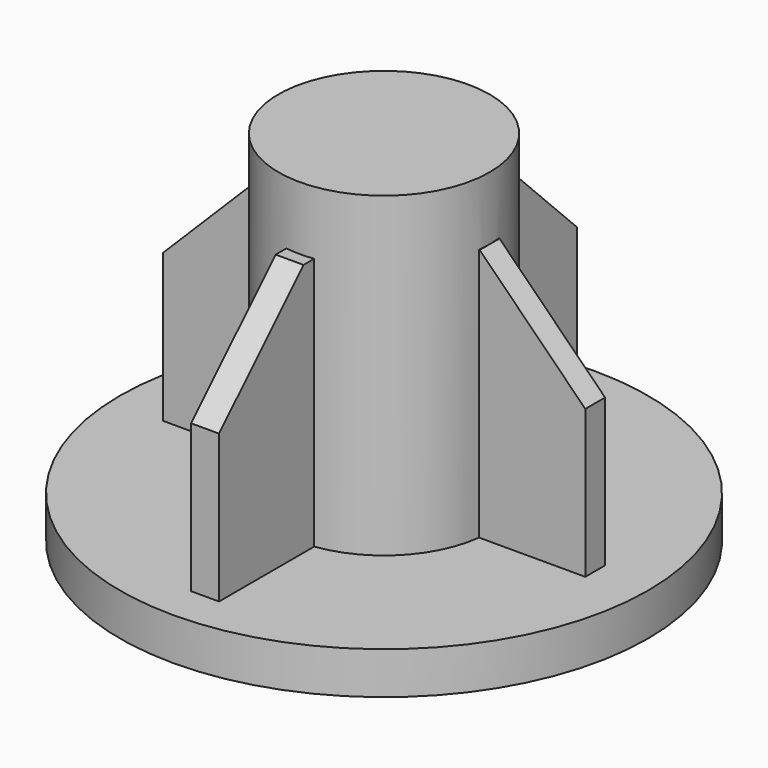
from build123d import *

# Parameters (mm, degrees)
F0_R     = 5
F2_DEPTH = 15
F1_W     = 9.3396854261
F1_H     = 1.1709111985
F1_W_2   = 1.3206291478
F1_H_2   = 10.0037873136
F3_DEPTH = 12
F4_SIZE  = 4.99999
F5_R     = 12.5
F6_DEPTH = 2


# Not quite as in the source:
# - a fillet or chamfer is up to 0.001 mm smaller than in the source, because OpenCascade refuses the exact size


with BuildPart() as f2:
    # F0 (on Top) → F2 (new body)
    with BuildSketch(Plane.XY):
        Circle(F0_R)
    extrude(amount=F2_DEPTH)

    # F1 (on Top) → F3 (join)
    with BuildSketch(Plane.XY):
        with Locations((5.330157287, 0)):
            Rectangle(F1_W, F1_H)
        with Locations((-5.330157287, 0)):
            Rectangle(F1_W, F1_H)
        with Locations((0, 5.587349256)):
            Rectangle(F1_W_2, F1_H_2)
        with Locations((0, -5.587349256)):
            Rectangle(F1_W_2, F1_H_2)
    extrude(amount=F3_DEPTH)

    # F4 (size 5 in the source; OpenCascade refuses exactly that, so slightly less here)
    f4_edges = [f2.edges().sort_by_distance(p)[0] for p in [
        (0, 10.589243, 12),
        (10, 0, 12),
        (0, -10.589243, 12),
        (-10, 0, 12),
    ]]
    chamfer(f4_edges, length=F4_SIZE)

    # F5 (on Top) → F6 (join)
    with BuildSketch(Plane.XY):
        Circle(F5_R)
    extrude(amount=-F6_DEPTH)


solid = f2.part
